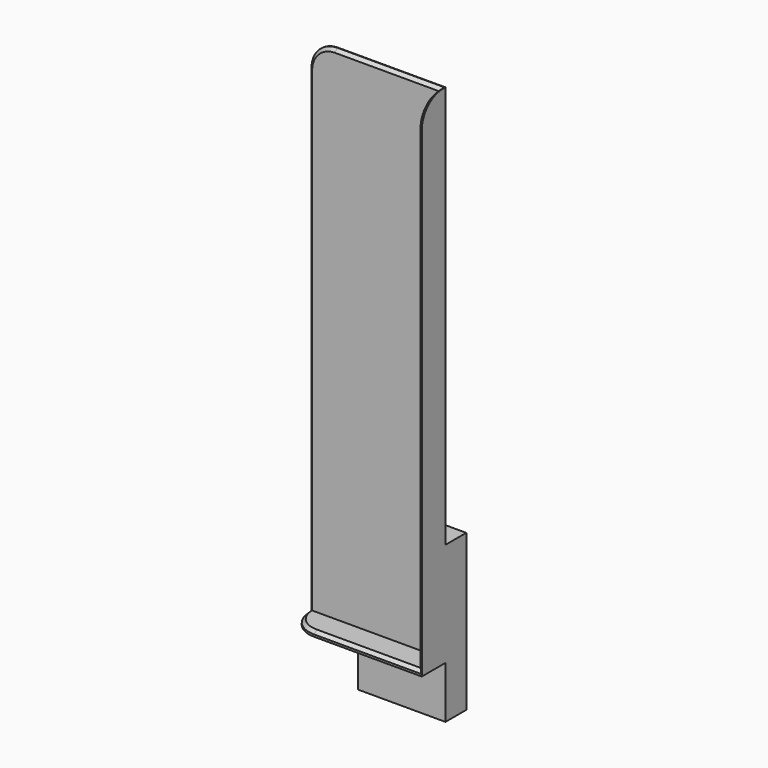
from build123d import *

# Parameters (mm, degrees)
F0_W        = 63.5
F0_H        = 247.65
F1_DEPTH    = 1.778
F2_W        = 63.5
F2_H        = 2.54
F3_DEPTH    = 12.7
F4_W        = 14.478
F4_H        = 247.65
F5_DEPTH    = 1.778
F6_W        = 42.672
F6_H        = 76.2
F7_DEPTH    = 12.7
F8_R        = 12.7
F9_R        = 12.7
F10_C1_SIZE = 1.524
F10_C2_SIZE = 1.524
F10_C3_SIZE = 1.5236


# Not quite as in the source:
# - a fillet or chamfer is up to 0.001 mm smaller than in the source, because OpenCascade refuses the exact size


with BuildPart() as f1:
    # F0 (on Front) → F1 (new body)
    with BuildSketch(Plane.XZ):
        with Locations((31.75, 123.825)):
            Rectangle(F0_W, F0_H)
    extrude(amount=F1_DEPTH)

    # F2 (on face) → F3 (join)
    with BuildSketch(Plane.XZ.offset(1.778)):
        with Locations((31.75, 1.27)):
            Rectangle(F2_W, F2_H)
    extrude(amount=F3_DEPTH)

    # F4 (on face) → F5 (join)
    with BuildSketch(Plane.YZ.offset(63.5)):
        with Locations((-7.239, 123.825)):
            Rectangle(F4_W, F4_H)
    extrude(amount=F5_DEPTH)

    # F6 (on face) → F7 (join)
    with BuildSketch(Plane(origin=(0, 0, 0), x_dir=(-1, 0, 0), z_dir=(0, 1, 0))):
        with Locations((-43.942, 12.7)):
            Rectangle(F6_W, F6_H)
    extrude(amount=F7_DEPTH)

    # F8
    f8_edges = [f1.edges().sort_by_distance(p)[0] for p in [
        (0, -0.889, 247.65),
        (64.389, -14.478, 247.65),
    ]]
    fillet(f8_edges, radius=F8_R)

    # F9
    f9_edges = [f1.edges().sort_by_distance(p)[0] for p in [
        (0, -14.478, 1.27),
    ]]
    fillet(f9_edges, radius=F9_R)

    # F10: chamfer of 1.524 on 3 edges, made by hand

    # F10_c1
    f10_c1_edges = [f1.edges().sort_by_distance(p)[0] for p in [
        (0, -1.778, 118.745),
        (3.7197438789, -1.778, 243.9302561211),
        (38.1, -1.778, 247.65),
    ]]
    chamfer(f10_c1_edges, length=F10_C1_SIZE)

    # F10_c2
    f10_c2_edges = [f1.edges().sort_by_distance(p)[0] for p in [
        (3.7197438789, -10.7582561211, 2.54),
        (38.1, -14.478, 2.54),
    ]]
    chamfer(f10_c2_edges, length=F10_C2_SIZE)

    # F10_c3 (size 1.524 in the source; OpenCascade refuses exactly that, so slightly less here)
    f10_c3_edges = [f1.edges().sort_by_distance(p)[0] for p in [
        (63.5, -14.478, 118.745),
        (63.5, -10.7582561211, 243.9302561211),
    ]]
    chamfer(f10_c3_edges, length=F10_C3_SIZE)


solid = f1.part
